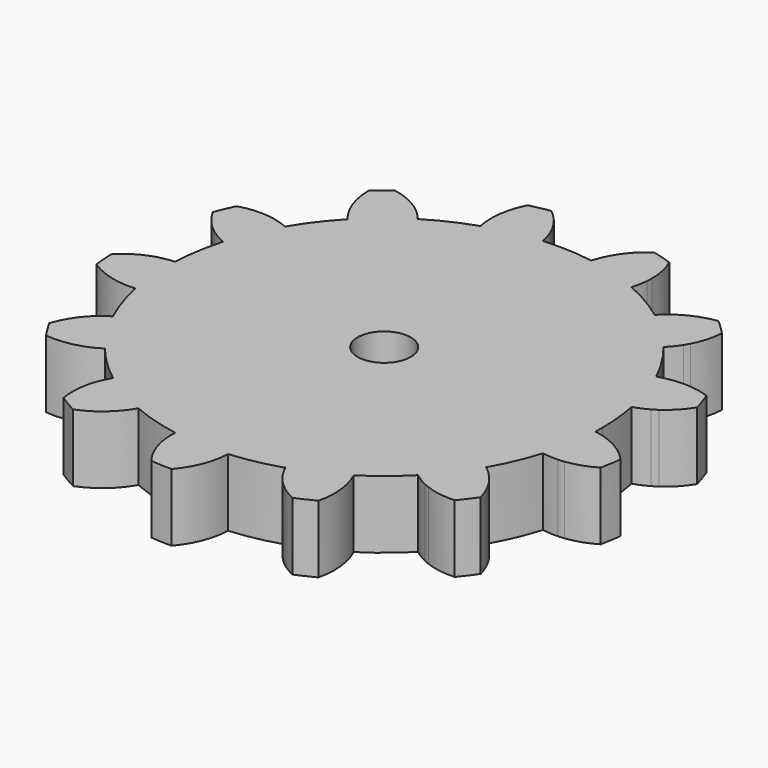
from build123d import *

# Parameters (mm, degrees)
F1_DEPTH = 6.35
F2_COUNT = 13
F3_R     = 2.5
F4_DEPTH = 25.4


with BuildPart() as f1:
    # F0 (on Top) → F1 (new body)
    with BuildSketch(Plane.XY):
        with BuildLine():
            ThreePointArc((7.9296197565, 23.5951858335), (6.9911317973, 23.8900761864), (6.0417249702, 24.1476546146))
            ThreePointArc((6.0417249702, 24.1476546146), (4.3226425573, 22.4330749308), (3.2648662162, 20.2476374354))
            ThreePointArc((3.2648662162, 20.2476374354), (5.7837443287, 19.6767495961), (8.2108987358, 18.7938105523))
            ThreePointArc((8.2108987358, 18.7938105523), (8.3954934616, 19.5156536929), (8.4994507341, 20.2534379554))
            ThreePointArc((8.4994507341, 20.2534379554), (8.5176465567, 20.5391701676), (8.5237154667, 20.8254168329))
            ThreePointArc((8.5237154667, 20.8254168329), (8.373521449, 22.2418004346), (7.9296197565, 23.5951858335))
        make_face()
        with BuildLine():
            ThreePointArc((4.0264902572, 14.4598933509), (-1.7431476836, 15.057566034), (-4.9211585336, 19.9100068261))
            ThreePointArc((-4.9211585336, 19.9100068261), (-12.6431262329, -16.1486077476), (20.5091729021, 0))
            ThreePointArc((20.5091729021, 0), (19.2415803806, 7.0984334598), (15.5954927821, 13.3194135761))
            ThreePointArc((15.5954927821, 13.3194135761), (9.5256046991, 10.9946956396), (4.0264902572, 14.4598933509))
        make_face()
        with BuildLine():
            ThreePointArc((3.2648662162, 20.2476374354), (-0.8451772993, 20.4917507417), (-4.9211585336, 19.9100068261))
            ThreePointArc((-4.9211585336, 19.9100068261), (-1.7431476836, 15.057566034), (4.0264902572, 14.4598933509))
            ThreePointArc((4.0264902572, 14.4598933509), (3.0384725246, 17.2738616412), (3.2648662162, 20.2476374354))
        make_face()
        with BuildLine():
            ThreePointArc((4.0264902572, 14.4598933509), (9.5256046991, 10.9946956396), (15.5954927821, 13.3194135761))
            ThreePointArc((15.5954927821, 13.3194135761), (12.2138579016, 16.4756744411), (8.2108987358, 18.7938105523))
            ThreePointArc((8.2108987358, 18.7938105523), (6.6287005247, 16.1344397874), (4.0264902572, 14.4598933509))
        make_face()
        with BuildLine():
            ThreePointArc((8.2108987358, 18.7938105523), (5.7837443287, 19.6767495961), (3.2648662162, 20.2476374354))
            ThreePointArc((3.2648662162, 20.2476374354), (3.0384725246, 17.2738616412), (4.0264902572, 14.4598933509))
            ThreePointArc((4.0264902572, 14.4598933509), (6.6287005247, 16.1344397874), (8.2108987358, 18.7938105523))
        make_face()
    extrude(amount=F1_DEPTH)

    # F2: F1 ×13 about axis
    f2_axis = Axis((0, 0, 6.35), (0, 0, 1))


with BuildPart() as f1_1:
    add(f1.part)
    for i in range(1, F2_COUNT):
        add(f1.part.rotate(f2_axis, i * 360 / F2_COUNT))

    # F3 (on face) → F4 (cut)
    with BuildSketch(Plane.XY.offset(6.35)):
        Circle(F3_R)
    extrude(amount=-F4_DEPTH, mode=Mode.SUBTRACT)


solid = f1_1.part
